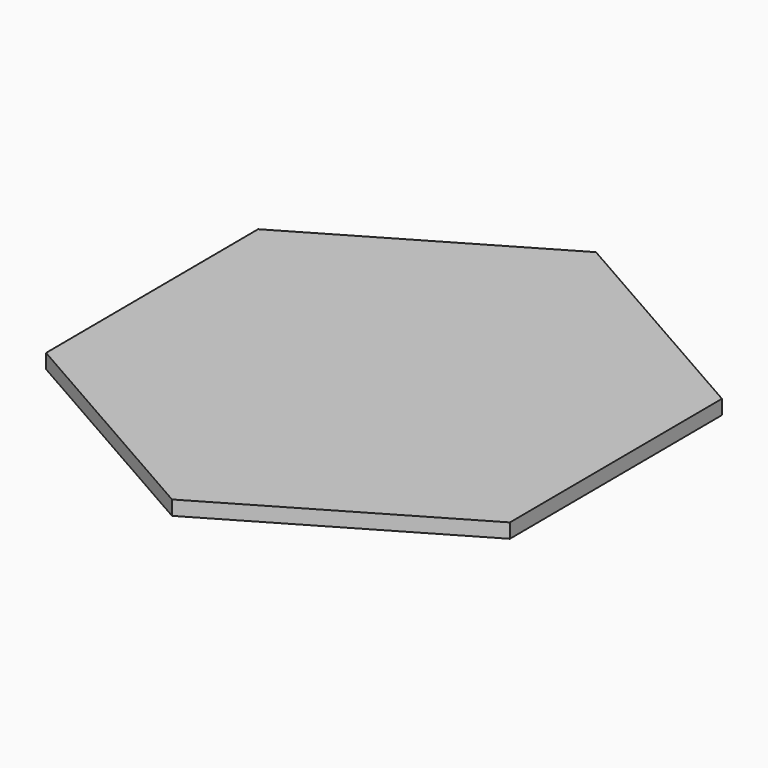
from build123d import *

# Parameters (mm, degrees)
F1_DEPTH = 3.175


# Not quite as in the source:
# - a length typed as a fraction of an inch, garbled in the dataset ("3 / 203.2 mm" for 3/8 in), is restored


with BuildPart() as f1:
    # F0 (on Top) → F1 (new body)
    with BuildSketch(Plane.XY):
        Polygon((-0.2999186872, 58.658020612), (-50.9492953293, 29.0692731038), (-50.6493766421, -29.5887475082), (0.2999186872, -58.658020612), (50.9492953293, -29.0692731038), (50.6493766421, 29.5887475082), align=None)
    extrude(amount=F1_DEPTH)


solid = f1.part
